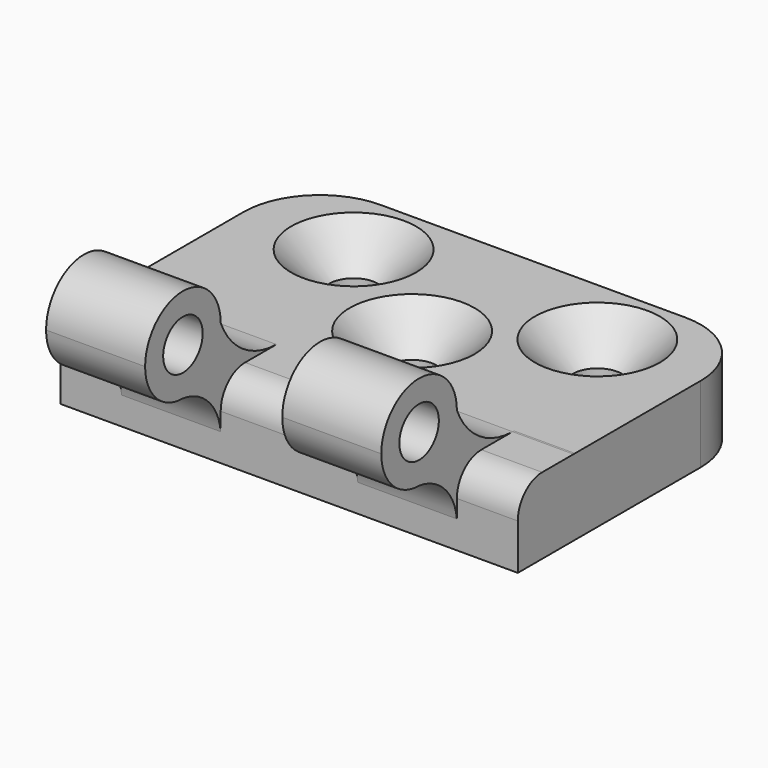
from build123d import *

# Parameters (mm, degrees)
F0_W      = 30
F0_H      = 20
F0_R      = 1.6
F1_DEPTH  = 5
F3_DEPTH  = 30
F7_DEPTH  = 7
F9_DEPTH  = 7
F10_SIZE  = 2.5
F11_R     = 5
F12_R     = 1.6200998357
F13_DEPTH = 30.001
F14_R     = 2
F17_DEPTH = 9


with BuildPart() as f1:
    # F0 (on Top) → F1 (new body)
    with BuildSketch(Plane.XY):
        Rectangle(F0_W, F0_H)
        with Locations((-8, 5.2767994255)):
            Circle(F0_R, mode=Mode.SUBTRACT)
        with Locations((0, 0.0767994255)):
            Circle(F0_R, mode=Mode.SUBTRACT)
        with Locations((8, 5.2767994255)):
            Circle(F0_R, mode=Mode.SUBTRACT)
    extrude(amount=F1_DEPTH)

    # F2 (on face) → F3 (join, through all)
    with BuildSketch(Plane(origin=(-15, 0, 0), x_dir=(0, -1, 0), z_dir=(-1, 0, 0))):
        with BuildLine():
            ThreePointArc((13.1, 5), (15.2920310217, 5.9079689783), (16.2, 8.1))
            ThreePointArc((16.2, 8.1), (13.1, 11.2), (10, 8.1))
            ThreePointArc((10, 8.1), (10.9079689783, 5.9079689783), (13.1, 5))
        make_face()
        with BuildLine():
            ThreePointArc((13.1, 5), (10.9079689783, 5.9079689783), (10, 8.1))
            ThreePointArc((10, 8.1), (8.1808280522, 5.8625059643), (5.4291286506, 5))
            Line((5.4291286506, 5), (10, 5))
            Line((10, 5), (10, 1.816622098))
            ThreePointArc((10, 1.816622098), (10.998268655, 3.9455916428), (13.1, 5))
        make_face()
    extrude(amount=-F3_DEPTH)

    # F6 (on offset) → F7 (cut)
    with BuildSketch(Plane.YZ.offset(11)):
        with BuildLine():
            ThreePointArc((-13.1, 5), (-10.9079689783, 5.9079689783), (-10, 8.1))
            ThreePointArc((-10, 8.1), (-15.2920310217, 10.2920310217), (-13.1, 5))
        make_face()
        with BuildLine():
            ThreePointArc((-5.4291286506, 5), (-8.1808280522, 5.8625059643), (-10, 8.1))
            ThreePointArc((-10, 8.1), (-10.9079689783, 5.9079689783), (-13.1, 5))
            ThreePointArc((-13.1, 5), (-10.998268655, 3.9455916428), (-10, 1.816622098))
            Line((-10, 1.816622098), (-10, 5))
            Line((-10, 5), (-5.4291286506, 5))
        make_face()
        with BuildLine():
            Line((-5.3136004135, 5), (-5.4291286506, 5))
            ThreePointArc((-5.4291286506, 5), (-5.371364532, 4.9996666743), (-5.3136004135, 5))
        make_face()
    extrude(amount=F7_DEPTH, mode=Mode.SUBTRACT)

    # F8 (on offset) → F9 (cut)
    with BuildSketch(Plane(origin=(-11, 0, 0), x_dir=(0, -1, 0), z_dir=(-1, 0, 0))):
        with BuildLine():
            ThreePointArc((13.1, 5), (15.2920310217, 5.9079689783), (16.2, 8.1))
            ThreePointArc((16.2, 8.1), (13.1, 11.2), (10, 8.1))
            ThreePointArc((10, 8.1), (10.9079689783, 5.9079689783), (13.1, 5))
        make_face()
        with BuildLine():
            ThreePointArc((5.3136004135, 5), (5.371364532, 4.9996666743), (5.4291286506, 5))
            Line((5.4291286506, 5), (5.3136004135, 5))
        make_face()
        with BuildLine():
            ThreePointArc((13.1, 5), (10.9079689783, 5.9079689783), (10, 8.1))
            ThreePointArc((10, 8.1), (8.1808280522, 5.8625059643), (5.4291286506, 5))
            Line((5.4291286506, 5), (10, 5))
            Line((10, 5), (10, 1.816622098))
            ThreePointArc((10, 1.816622098), (10.998268655, 3.9455916428), (13.1, 5))
        make_face()
    extrude(amount=F9_DEPTH, mode=Mode.SUBTRACT)

    # F10
    f10_edges = [f1.edges().sort_by_distance(p)[0] for p in [
        (-9.6, 5.276799, 5),
        (-1.6, 0.076799, 5),
        (6.4, 5.276799, 5),
    ]]
    chamfer(f10_edges, length=F10_SIZE)

    # F11
    f11_edges = [f1.edges().sort_by_distance(p)[0] for p in [
        (-15, 10, 2.5),
        (15, 10, 2.5),
    ]]
    fillet(f11_edges, radius=F11_R)

    # F12 (on face) → F13 (cut, through all)
    with BuildSketch(Plane(origin=(-15, 0, 0), x_dir=(0, -1, 0), z_dir=(-1, 0, 0))):
        with Locations((13.1, 8.1)):
            Circle(F12_R)
    extrude(amount=-F13_DEPTH, mode=Mode.SUBTRACT)

    # F14
    f14_edges = [f1.edges().sort_by_distance(p)[0] for p in [
        (-13, -10, 5),
        (13, -10, 5),
    ]]
    fillet(f14_edges, radius=F14_R)

    # F16 (on offset) → F17 (cut)
    with BuildSketch(Plane(origin=(-4.5, 0, 0), x_dir=(0, -1, 0), z_dir=(-1, 0, 0))):
        with BuildLine():
            ThreePointArc((10, 1.816622098), (10.998268655, 3.9455916428), (13.1, 5))
            ThreePointArc((13.1, 5), (15.2920310217, 10.2920310217), (10, 8.1))
            ThreePointArc((10, 8.1), (8.1808280522, 5.8625059643), (5.4291286506, 5))
            Line((5.4291286506, 5), (8, 5))
            ThreePointArc((8, 5), (9.4142135624, 4.4142135624), (10, 3))
            Line((10, 3), (10, 1.816622098))
        make_face()
    extrude(amount=-F17_DEPTH, mode=Mode.SUBTRACT)


solid = f1.part
